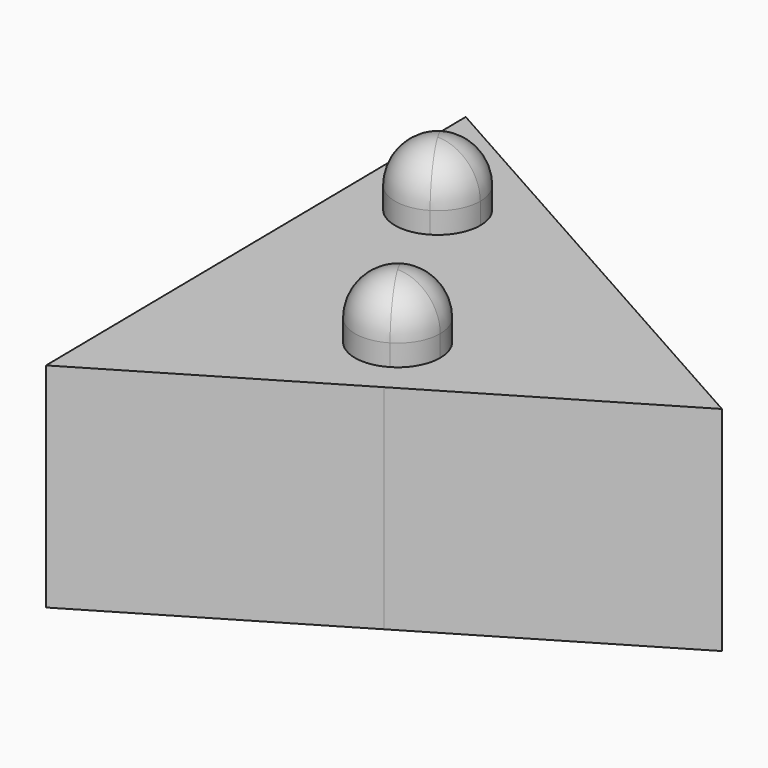
from build123d import *

# Parameters (mm, degrees)
F1_DEPTH = 50
F2_DEPTH = 65
F3_R     = 10


with BuildPart() as f1:
    # F0 (on Top) → F1 (new body)
    with BuildSketch(Plane.XY):
        with BuildLine():
            Line((18.428938438, -31.0235001472), (72.1632169215, 0.8963575571))
            Line((72.1632169215, 0.8963575571), (-36.8578768761, 62.0470002943))
            Line((-36.8578768761, 62.0470002943), (-22.982297547, 38.6886805081))
            ThreePointArc((-22.982297547, 38.6886805081), (-12.9289992244, 38.7823343206), (-7.8751203144, 30.0911959508))
            ThreePointArc((-7.8751203144, 30.0911959508), (-9.1839819445, 25.1450748608), (-12.7679430817, 21.4937113934))
            Line((-12.7679430817, 21.4937113934), (0, 0))
            Line((0, 0), (4.1072919863, -6.9142655162))
            ThreePointArc((4.1072919863, -6.9142655162), (14.160590309, -6.8206117038), (19.214469219, -15.5117500736))
            ThreePointArc((19.214469219, -15.5117500736), (17.9056075888, -20.4578711635), (14.3216464517, -24.1092346309))
            Line((14.3216464517, -24.1092346309), (18.428938438, -31.0235001472))
        make_face()
        with BuildLine():
            Line((-35.3053400455, -62.9433578514), (18.428938438, -31.0235001472))
            Line((18.428938438, -31.0235001472), (14.3216464517, -24.1092346309))
            ThreePointArc((14.3216464517, -24.1092346309), (0.6169846617, -20.6189273063), (4.1072919863, -6.9142655162))
            Line((4.1072919863, -6.9142655162), (0, 0))
            Line((0, 0), (-12.7679430817, 21.4937113934))
            ThreePointArc((-12.7679430817, 21.4937113934), (-26.4726048717, 24.9840187181), (-22.982297547, 38.6886805081))
            Line((-22.982297547, 38.6886805081), (-36.8578768761, 62.0470002943))
            Line((-36.8578768761, 62.0470002943), (-35.3053400455, -62.9433578514))
        make_face()
    extrude(amount=F1_DEPTH)

    # F0 (on Top) → F2 (join)
    with BuildSketch(Plane.XY):
        with BuildLine():
            ThreePointArc((-7.8751203144, 30.0911959508), (-12.9289992244, 38.7823343206), (-22.982297547, 38.6886805081))
            Line((-22.982297547, 38.6886805081), (-12.7679430817, 21.4937113934))
            ThreePointArc((-12.7679430817, 21.4937113934), (-9.1839819445, 25.1450748608), (-7.8751203144, 30.0911959508))
        make_face()
        with BuildLine():
            Line((-12.7679430817, 21.4937113934), (-22.982297547, 38.6886805081))
            ThreePointArc((-22.982297547, 38.6886805081), (-26.4726048717, 24.9840187181), (-12.7679430817, 21.4937113934))
        make_face()
        with BuildLine():
            ThreePointArc((4.1072919863, -6.9142655162), (0.6169846617, -20.6189273063), (14.3216464517, -24.1092346309))
            Line((14.3216464517, -24.1092346309), (4.1072919863, -6.9142655162))
        make_face()
        with BuildLine():
            Line((4.1072919863, -6.9142655162), (14.3216464517, -24.1092346309))
            ThreePointArc((14.3216464517, -24.1092346309), (17.9056075888, -20.4578711635), (19.214469219, -15.5117500736))
            ThreePointArc((19.214469219, -15.5117500736), (14.160590309, -6.8206117038), (4.1072919863, -6.9142655162))
        make_face()
    extrude(amount=F2_DEPTH)

    # F3
    f3_edges = [f1.edges().sort_by_distance(p)[0] for p in [
        (-27.87512, 30.091196, 65),
        (4.107292, -6.914266, 65),
    ]]
    fillet(f3_edges, radius=F3_R)


solid = f1.part
